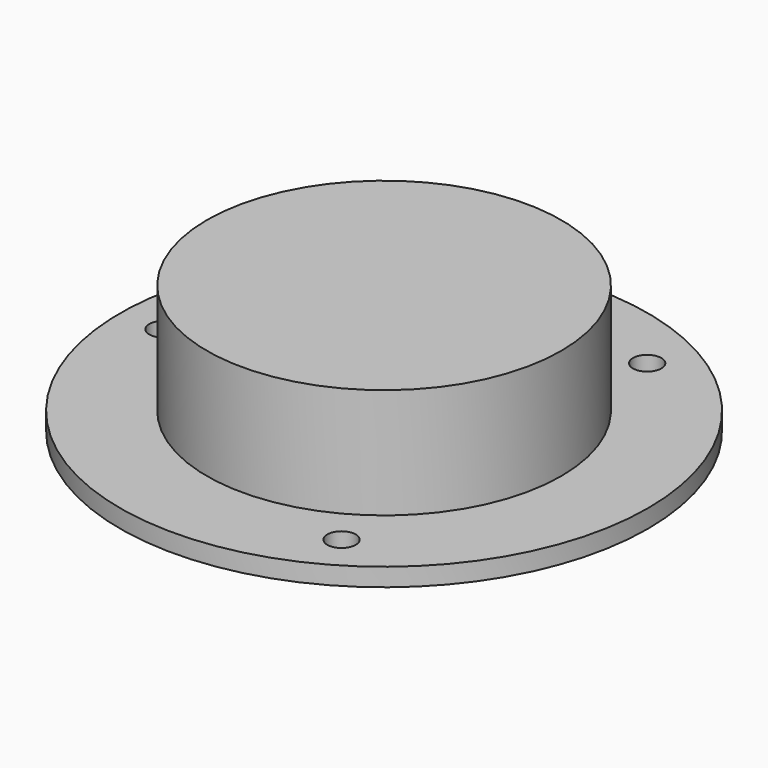
from build123d import *

# Parameters (mm, degrees)
F1_DEPTH = 18.034
F0_R     = 1.9939
F2_DEPTH = 2.54


# Not quite as in the source:
# - a feature names something its author has since deleted; it is built from what else it names


with BuildPart() as f1:
    # F0 (on Top) → F1 (new body)
    with BuildSketch(Plane.XY):
        with BuildLine():
            ThreePointArc((24.892, 0), (0, 24.892), (-24.892, 0))
            ThreePointArc((-24.892, 0), (0, -24.892), (24.892, 0))
        make_face()
    extrude(amount=F1_DEPTH)

    # F0 (on Top) → F2 (join)
    with BuildSketch(Plane.XY):
        with BuildLine():
            ThreePointArc((-37.084, 0), (0, -37.084), (37.084, 0))
            ThreePointArc((37.084, 0), (0, 37.084), (-37.084, 0))
        make_face()
        with Locations((15.494, -26.8363952125)):
            Circle(F0_R, mode=Mode.SUBTRACT)
        with BuildLine():
            ThreePointArc((-28.9941, 0), (-30.988, -1.9939), (-32.9819, 0))
            ThreePointArc((-32.9819, 0), (-30.988, 1.9939), (-28.9941, 0))
        make_face(mode=Mode.SUBTRACT)
        with BuildLine():
            ThreePointArc((24.892, 0), (0, -24.892), (-24.892, 0))
            ThreePointArc((-24.892, 0), (0, 24.892), (24.892, 0))
        make_face(mode=Mode.SUBTRACT)
        with Locations((15.494, 26.8363952125)):
            Circle(F0_R, mode=Mode.SUBTRACT)
    extrude(amount=F2_DEPTH)


solid = f1.part
